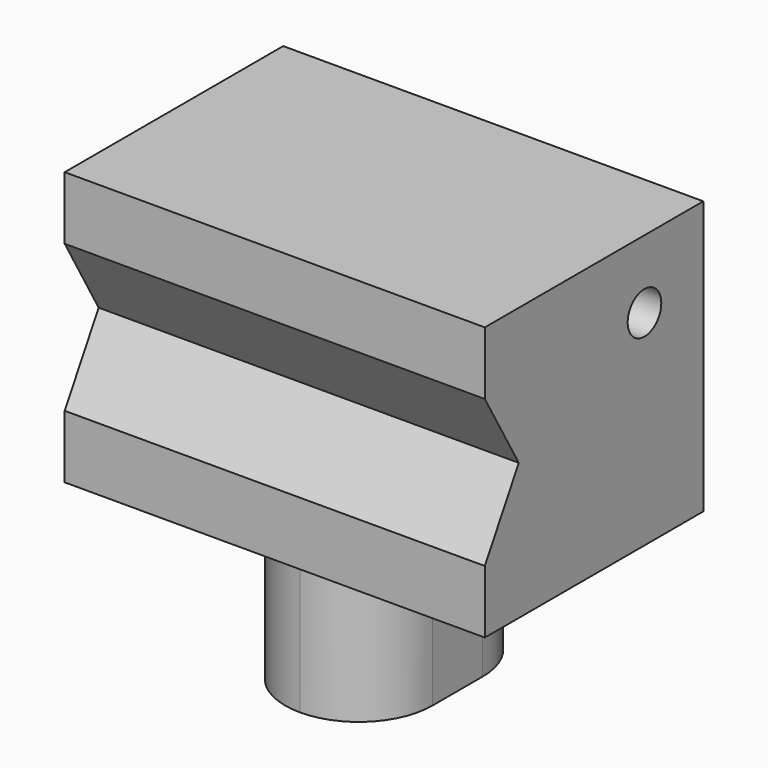
from build123d import *

# Parameters (mm, degrees)
F1_DEPTH  = 20
F2_W      = 14
F2_H      = 20
F3_DEPTH  = 14
F4_R      = 6.99999
F6_D      = 13
F6_DEPTH  = 16
F6_TIP    = 3.9055940237
F7_R      = 2
F8_DEPTH  = 20
F10_D     = 4.2
F10_DEPTH = 14.6
F10_TIP   = 1.2618073


# Not quite as in the source:
# - a fillet or chamfer is up to 0.001 mm smaller than in the source, because OpenCascade refuses the exact size


with BuildPart() as f1:
    # F0 (on Right) → F1 (new body, symmetric)
    with BuildSketch(Plane.YZ):
        Polygon((-13, -13), (13, -13), (13, 13), (-13, 13), (-13, 7), (-8.9585481157, 0), (-13, -7), align=None)
    extrude(amount=F1_DEPTH, both=True)

    # F2 (on face) → F3 (join)
    with BuildSketch(Plane(origin=(0, 0, -13), x_dir=(1, 0, 0), z_dir=(0, 0, -1))):
        Rectangle(F2_W, F2_H)
    extrude(amount=F3_DEPTH)

    # F4 (radius 7 in the source; OpenCascade refuses exactly that, so slightly less here)
    f4_edges = [f1.edges().sort_by_distance(p)[0] for p in [
        (7, -10, -20),
        (-7, -10, -20),
        (7, 10, -20),
        (-7, 10, -20),
    ]]
    fillet(f4_edges, radius=F4_R)

    # F6
    with Locations(Plane(origin=(0, 13, 0), x_dir=(-1, 0, 0), z_dir=(0, 1, 0))):
        with Locations((0, 0)):
            Hole(F6_D / 2, depth=F6_DEPTH)
            with Locations((0, 0, -(F6_DEPTH + F6_TIP / 2))):  # 118° drill point
                Cone(0, F6_D / 2, F6_TIP, mode=Mode.SUBTRACT)

    # F7 (on Right) → F8 (cut, symmetric)
    with BuildSketch(Plane.YZ):
        with Locations((6, 6.5)):
            Circle(F7_R)
    extrude(amount=F8_DEPTH, both=True, mode=Mode.SUBTRACT)

    # F10
    with Locations(Plane(origin=(0, 0, -27), x_dir=(1, 0, 0), z_dir=(0, 0, -1))):
        with Locations((0, 0)):
            Hole(F10_D / 2, depth=F10_DEPTH)
            with Locations((0, 0, -(F10_DEPTH + F10_TIP / 2))):  # 118° drill point
                Cone(0, F10_D / 2, F10_TIP, mode=Mode.SUBTRACT)


solid = f1.part
